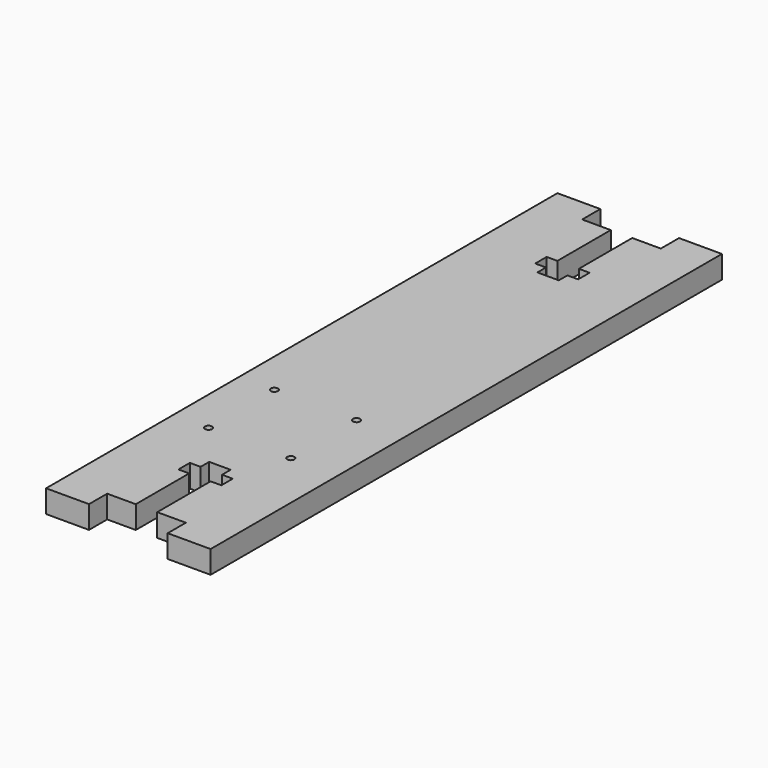
from build123d import *

# Parameters (mm, degrees)
F0_R     = 0.5
F1_DEPTH = 3.175


# Not quite as in the source:
# - a length typed as a fraction of an inch, garbled in the dataset ("3 / 203.2 mm" for 3/8 in), is restored


with BuildPart() as f1:
    # F0 (on Top) → F1 (new body)
    with BuildSketch(Plane.XY):
        Polygon((-34.3393906951, 49.0726131633), (-37.3393906951, 49.0726131633), (-37.3393906951, 50.5726131633), (-38.8393906951, 50.5726131633), (-38.8393906951, 52.5726131633), (-37.3393906951, 52.5726131633), (-37.3393906951, 61.8976131633), (-41.3393906951, 61.8976131633), (-41.3393906951, 65.0726131633), (-47.3393906951, 65.0726131633), (-47.3393906951, 61.8976131633), (-47.3393906951, -21.1023868367), (-47.3393906951, -24.2773868367), (-41.3393906951, -24.2773868367), (-41.3393906951, -21.1023868367), (-37.3393906951, -21.1023868367), (-37.3393906951, -11.7773868367), (-38.8393906951, -11.7773868367), (-38.8393906951, -9.7773868367), (-37.3393906951, -9.7773868367), (-37.3393906951, -8.2773868367), (-34.3393906951, -8.2773868367), (-34.3393906951, -9.7773868367), (-32.8393906951, -9.7773868367), (-32.8393906951, -11.7773868367), (-34.3393906951, -11.7773868367), (-34.3393906951, -21.1023868367), (-30.3393906951, -21.1023868367), (-30.3393906951, -24.2773868367), (-24.3393906951, -24.2773868367), (-24.3393906951, -21.1023868367), (-24.3393906951, 61.8976131633), (-24.3393906951, 65.0726131633), (-30.3393906951, 65.0726131633), (-30.3393906951, 61.8976131633), (-34.3393906951, 61.8976131633), (-34.3393906951, 52.5726131633), (-32.8393906951, 52.5726131633), (-32.8393906951, 50.5726131633), (-34.3393906951, 50.5726131633), align=None)
        with Locations((-42.4286872149, -2.0273868367)):
            Circle(F0_R, mode=Mode.SUBTRACT)
        with Locations((-42.4286872149, 9.4726131633)):
            Circle(F0_R, mode=Mode.SUBTRACT)
        with Locations((-30.9286872149, -2.0273868367)):
            Circle(F0_R, mode=Mode.SUBTRACT)
        with Locations((-30.9286872149, 9.4726131633)):
            Circle(F0_R, mode=Mode.SUBTRACT)
    extrude(amount=F1_DEPTH)


solid = f1.part
